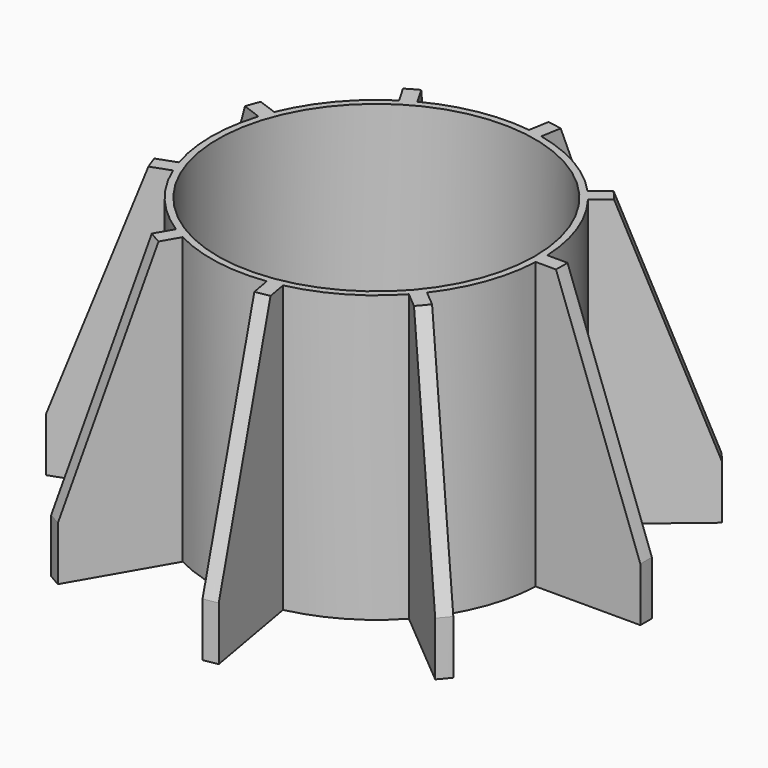
from build123d import *

# Parameters (mm, degrees)
F0_R            = 63.5
F0_R_2          = 37.3126
F1_DEPTH        = 67.231133
F5_DEPTH        = 67.231133
F5_COPIES_COUNT = 9
F6_COUNT        = 9
F6_ANGLE        = 320


# Not quite as in the source:
# - a pattern or mirror of a feature is missing from the dataset's text; its kind, count and spacing are read off the source's solid


with BuildPart() as f1:
    # F0 (on Top) → F1 (new body)
    with BuildSketch(Plane.XY):
        Circle(F0_R)
        Circle(F0_R_2, mode=Mode.SUBTRACT)
    extrude(amount=F1_DEPTH)

    # F2 (on Front) → F3 (revolve, cut)
    with BuildSketch(Plane.XZ):
        Polygon((43.6626, 110.893733), (43.6626, 67.231133), (63.5, 12.7), (63.5, 0), (107.1626, 0), (107.1626, 110.893733), align=None)
    revolve(axis=Axis((0, 0, 67.231133), (0, 0, 1)), mode=Mode.SUBTRACT)

    # F4 (on face) → F5 (cut, through all)
    with BuildSketch(Plane(origin=(0, 0, 0), x_dir=(1, 0, 0), z_dir=(0, 0, -1))):
        with BuildLine():
            ThreePointArc((-37.0996847558, -11.6974856713), (-38.9001, 0), (-37.0996847558, 11.6974856713))
            Line((-37.0996847558, 11.6974856713), (-60.2295137998, 20.116054967))
            ThreePointArc((-60.2295137998, 20.116054967), (-63.5, 0), (-60.2295137998, -20.116054967))
            Line((-60.2295137998, -20.116054967), (-37.0996847558, -11.6974856713))
        make_face()
    f5 = extrude(amount=-F5_DEPTH, mode=Mode.SUBTRACT)

    # F5_copies: F5 ×9 about axis
    f5_copies_axis = Axis((0, 0, 0), (0, 0, 1))
    for i in range(1, F5_COPIES_COUNT):
        add(f5.rotate(f5_copies_axis, i * 360 / F5_COPIES_COUNT), mode=Mode.SUBTRACT)

    # F6: F5 ×9 about axis
    f6_axis = Axis((0, 0, 67.231133), (0, 0, -1))
    for i in range(1, F6_COUNT):
        add(f5.rotate(f6_axis, i * F6_ANGLE / (F6_COUNT - 1)), mode=Mode.SUBTRACT)


solid = f1.part
